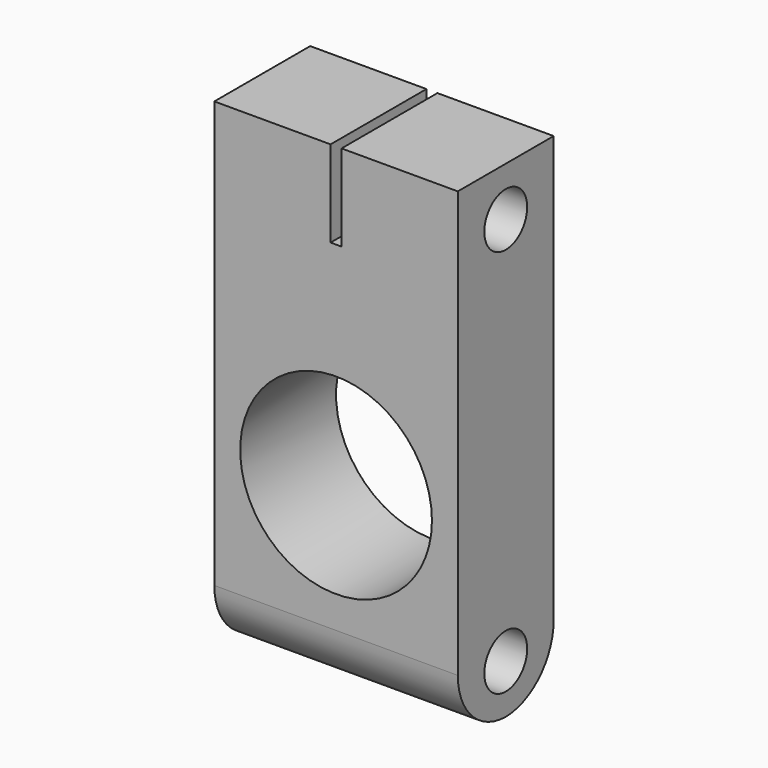
from build123d import *

# Parameters (mm, degrees)
F0_W         = 10.16
F0_H         = 20.32
F2_DEPTH     = 2.5
F1_R         = 4.0005
F3_DEPTH     = 4
F4_R         = 1.1176
F5_DEPTH     = 10.16
F6_W         = 0.4572
F6_H         = 5
F7_DEPTH     = 3.6068
F8_R         = 1.1176
F9_DEPTH     = 10.16
F10_T1_DEPTH = 22.86


# Not quite as in the source:
# - a fillet or chamfer that OpenCascade refuses, or shapes differently, is made with other operations: its cross-section is extruded or revolved along the edge and cut away or added


with BuildPart() as f2:
    # F0 (on Front) → F2 (new body, symmetric)
    with BuildSketch(Plane.XZ):
        Rectangle(F0_W, F0_H)
    extrude(amount=F2_DEPTH, both=True)

    # F1 (on face) → F3 (cut, symmetric)
    with BuildSketch(Plane.XZ):
        with Locations((0, -2.2881471086)):
            Circle(F1_R)
    extrude(amount=F3_DEPTH, both=True, mode=Mode.SUBTRACT)

    # F4 (on face) → F5 (cut)
    with BuildSketch(Plane.YZ.offset(5.08)):
        with Locations((0, -8.1131188199)):
            Circle(F4_R)
    extrude(amount=-F5_DEPTH, mode=Mode.SUBTRACT)

    # F6 (on face) → F7 (cut)
    with BuildSketch(Plane.XY.offset(10.16)):
        Rectangle(F6_W, F6_H)
    extrude(amount=-F7_DEPTH, mode=Mode.SUBTRACT)

    # F8 (on face) → F9 (cut)
    with BuildSketch(Plane.YZ.offset(5.08)):
        with Locations((0, 8.1132977634)):
            Circle(F8_R)
    extrude(amount=-F9_DEPTH, mode=Mode.SUBTRACT)

    # F10: fillet of radius 2.54 on 2 edges, made by hand

    # F10_s2 → F10_t1 (cut)
    with BuildSketch(Plane.YZ.offset(-11.43)):
        with BuildLine():
            ThreePointArc((-0.04, -10.16), (1.7560512242, -9.4160512242), (2.5, -7.62))
            Line((2.5, -7.62), (2.5, -10.16))
            Line((2.5, -10.16), (-0.04, -10.16))
        make_face()
        with BuildLine():
            ThreePointArc((0.04, -10.16), (-1.7560512242, -9.4160512242), (-2.5, -7.62))
            Line((-2.5, -7.62), (-2.5, -10.16))
            Line((-2.5, -10.16), (0.04, -10.16))
        make_face()
    extrude(amount=F10_T1_DEPTH, mode=Mode.SUBTRACT)


solid = f2.part
